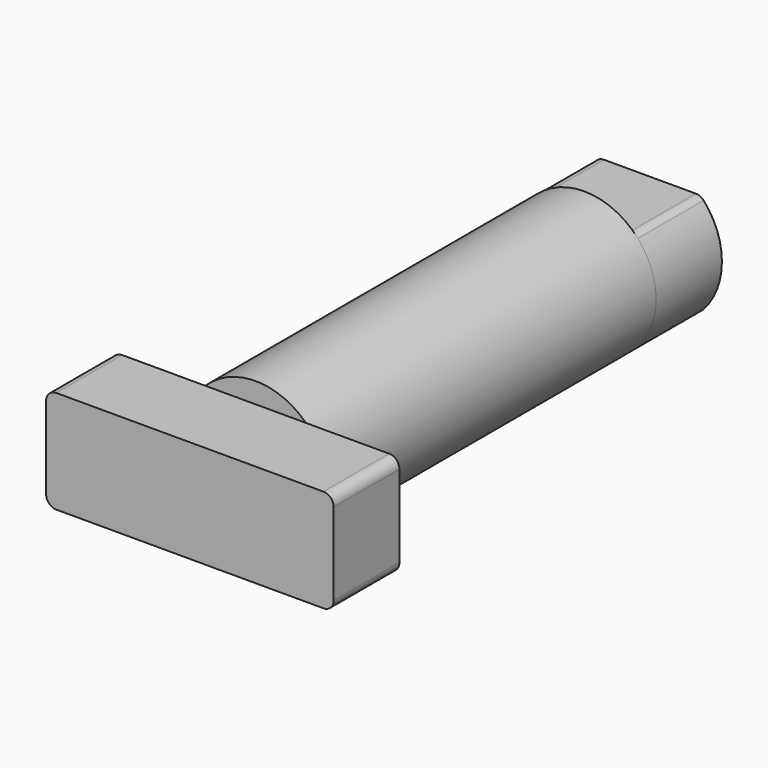
from build123d import *
from build123d import SkipClean  # not in build123d's __all__

# Parameters (mm, degrees)
F1_DEPTH    = 10
F3_DEPTH    = 4
F5_DEPTH    = 4
F6_R        = 0.5
F7_T1_DEPTH = 20
F7_T3_DEPTH = 4.5763046334


# Not quite as in the source:
# - a fillet or chamfer that OpenCascade refuses, or shapes differently, is made with other operations: its cross-section is extruded or revolved along the edge and cut away or added


with BuildPart() as f1:
    # F0 (on Front) → F1 (new body, symmetric)
    with BuildSketch(Plane.XZ):
        with BuildLine():
            Line((-2.4494897428, 0), (2.4494897428, 0))
            ThreePointArc((2.4494897428, 0), (0, 6), (-2.4494897428, 0))
        make_face()
    extrude(amount=F1_DEPTH, both=True)

    # F2 (on face) → F3 (join)
    with BuildSketch(Plane.XZ.offset(10)):
        with BuildLine():
            Line((-2.4494897428, 5), (-7, 5))
            Line((-7, 5), (-7, 0))
            Line((-7, 0), (-2.4494897428, 0))
            ThreePointArc((-2.4494897428, 0), (-3.5, 2.5), (-2.4494897428, 5))
        make_face()
        with BuildLine():
            Line((2.4494897428, 5), (-2.4494897428, 5))
            ThreePointArc((-2.4494897428, 5), (-3.5, 2.5), (-2.4494897428, 0))
            Line((-2.4494897428, 0), (2.4494897428, 0))
            ThreePointArc((2.4494897428, 0), (3.5, 2.5), (2.4494897428, 5))
        make_face()
        with BuildLine():
            Line((7, 5), (2.4494897428, 5))
            ThreePointArc((2.4494897428, 5), (3.5, 2.5), (2.4494897428, 0))
            Line((2.4494897428, 0), (7, 0))
            Line((7, 0), (7, 5))
        make_face()
    extrude(amount=F3_DEPTH)

    # F4 (on face) → F5 (join)
    with BuildSketch(Plane(origin=(0, 10, 0), x_dir=(-1, 0, 0), z_dir=(0, 1, 0))):
        with BuildLine():
            ThreePointArc((-2.4494897428, 5), (-3.5, 2.5), (-2.4494897428, 0))
            Line((-2.4494897428, 0), (2.4494897428, 0))
            ThreePointArc((2.4494897428, 0), (3.5, 2.5), (2.4494897428, 5))
            Line((2.4494897428, 5), (-2.4494897428, 5))
        make_face()
    extrude(amount=F5_DEPTH)

    # F6
    f6_edges = [f1.edges().sort_by_distance(p)[0] for p in [
        (7, -12, 5),
        (7, -12, 0),
        (-7, -12, 5),
        (-7, -12, 0),
    ]]
    fillet(f6_edges, radius=F6_R)

    # F7: fillet of radius 0.5 on 6 edges, made by hand

    # F7_s2 → F7_t1 (cut)
    with BuildSketch(Plane.XZ.offset(-10)):
        with BuildLine():
            ThreePointArc((2.2360679775, 0), (2.4401921227, 0.0435645354), (2.6087459737, 0.1666666667))
            ThreePointArc((2.6087459737, 0.1666666667), (2.5304903844, 0.0820218333), (2.4494897428, 0))
            Line((2.4494897428, 0), (2.2360679775, 0))
        make_face()
        with BuildLine():
            ThreePointArc((-2.2360679775, 0), (-2.4401921227, 0.0435645354), (-2.6087459737, 0.1666666667))
            ThreePointArc((-2.6087459737, 0.1666666667), (-2.5304903844, 0.0820218333), (-2.4494897428, 0))
            Line((-2.4494897428, 0), (-2.2360679775, 0))
        make_face()
    with SkipClean():  # cleaning this boolean's faces spoils the solid; the shape is the same uncleaned
        extrude(amount=F7_T1_DEPTH, mode=Mode.SUBTRACT)

    # F7_s4 → F7_t3 (cut)
    with BuildSketch(Plane.XZ.offset(-14.5763046334)):
        with BuildLine():
            ThreePointArc((2.2360679775, 0), (2.4401921227, 0.0435645354), (2.6087459737, 0.1666666667))
            ThreePointArc((2.6087459737, 0.1666666667), (2.5304903844, 0.0820218333), (2.4494897428, 0))
            Line((2.4494897428, 0), (2.2360679775, 0))
        make_face()
        with BuildLine():
            ThreePointArc((-2.2360679775, 0), (-2.4401921227, 0.0435645354), (-2.6087459737, 0.1666666667))
            ThreePointArc((-2.6087459737, 0.1666666667), (-2.5304903844, 0.0820218333), (-2.4494897428, 0))
            Line((-2.4494897428, 0), (-2.2360679775, 0))
        make_face()
        with BuildLine():
            ThreePointArc((2.6087459737, 4.8333333333), (2.4401921227, 4.9564354646), (2.2360679775, 5))
            Line((2.2360679775, 5), (2.4494897428, 5))
            ThreePointArc((2.4494897428, 5), (2.5304903844, 4.9179781667), (2.6087459737, 4.8333333333))
        make_face()
        with BuildLine():
            ThreePointArc((-2.6087459737, 4.8333333333), (-2.4401921227, 4.9564354646), (-2.2360679775, 5))
            Line((-2.2360679775, 5), (-2.4494897428, 5))
            ThreePointArc((-2.4494897428, 5), (-2.5304903844, 4.9179781667), (-2.6087459737, 4.8333333333))
        make_face()
    extrude(amount=F7_T3_DEPTH, mode=Mode.SUBTRACT)


solid = f1.part
